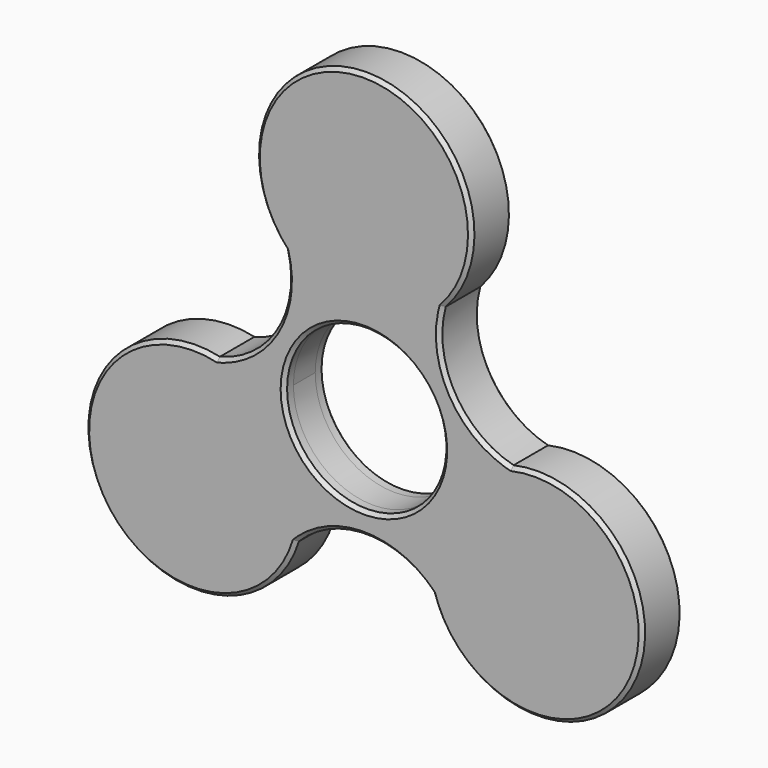
from build123d import *

# Parameters (mm, degrees)
F0_R        = 13.25
F0_R_2      = 11.1
F1_DEPTH    = 3
F2_START    = 1.9
F2_DEPTH    = 1.6
F3_START    = -1.9
F3_DEPTH    = 1.6
F5_D        = 22.2
F6_C1_SIZE  = 0.5
F6_C2_SIZE  = 0.5
F6_C3_SIZE  = 0.4999
F6_C4_SIZE  = 0.4999
F6_C5_SIZE  = 0.4999
F6_C6_SIZE  = 0.4999
F6_C7_SIZE  = 0.4996
F6_C8_SIZE  = 0.5
F6_C9_SIZE  = 0.4999
F6_C10_SIZE = 0.5
F6_C11_SIZE = 0.5
F6_C12_SIZE = 0.4999
F6_C13_SIZE = 0.4996
F6_C14_SIZE = 0.5


# Not quite as in the source:
# - a fillet or chamfer is up to 0.001 mm smaller than in the source, because OpenCascade refuses the exact size


with BuildPart() as f1:
    # F0 (on Front) → F1 (new body, symmetric)
    with BuildSketch(Plane.XZ):
        with BuildLine():
            ThreePointArc((20.4544666255, 0.9003555386), (12.301399045, 7.10221605), (11.0069640816, 17.2639099492))
            ThreePointArc((11.0069640816, 17.2639099492), (0, 42.4544321001), (-11.0069640816, 17.2639099492))
            ThreePointArc((-11.0069640816, 17.2639099492), (-12.301399045, 7.10221605), (-20.4544666255, 0.9003555386))
            ThreePointArc((-20.4544666255, 0.9003555386), (-36.7666167019, -21.22721605), (-9.4475025439, -18.1642654878))
            ThreePointArc((-9.4475025439, -18.1642654878), (0, -14.2044321001), (9.4475025439, -18.1642654878))
            ThreePointArc((9.4475025439, -18.1642654878), (36.7666167019, -21.22721605), (20.4544666255, 0.9003555386))
        make_face()
        with Locations((-23.7762356451, -13.72721605)):
            Circle(F0_R, mode=Mode.SUBTRACT)
        with Locations((23.7762356451, -13.72721605)):
            Circle(F0_R, mode=Mode.SUBTRACT)
        Circle(F0_R_2, mode=Mode.SUBTRACT)
        with Locations((0, 27.4544321001)):
            Circle(F0_R, mode=Mode.SUBTRACT)
    extrude(amount=F1_DEPTH, both=True)

    # F0 (on Front) → F2 (join)
    with BuildSketch(Plane.XZ.offset(F2_START)):
        with BuildLine():
            ThreePointArc((20.4544666255, 0.9003555386), (12.301399045, 7.10221605), (11.0069640816, 17.2639099492))
            ThreePointArc((11.0069640816, 17.2639099492), (0, 42.4544321001), (-11.0069640816, 17.2639099492))
            ThreePointArc((-11.0069640816, 17.2639099492), (-12.301399045, 7.10221605), (-20.4544666255, 0.9003555386))
            ThreePointArc((-20.4544666255, 0.9003555386), (-36.7666167019, -21.22721605), (-9.4475025439, -18.1642654878))
            ThreePointArc((-9.4475025439, -18.1642654878), (0, -14.2044321001), (9.4475025439, -18.1642654878))
            ThreePointArc((9.4475025439, -18.1642654878), (36.7666167019, -21.22721605), (20.4544666255, 0.9003555386))
        make_face()
        with Locations((-23.7762356451, -13.72721605)):
            Circle(F0_R, mode=Mode.SUBTRACT)
        with Locations((23.7762356451, -13.72721605)):
            Circle(F0_R, mode=Mode.SUBTRACT)
        Circle(F0_R_2, mode=Mode.SUBTRACT)
        with Locations((0, 27.4544321001)):
            Circle(F0_R, mode=Mode.SUBTRACT)
        with Locations((-23.7762356451, -13.72721605)):
            Circle(F0_R)
        with Locations((0, 27.4544321001)):
            Circle(F0_R)
        with Locations((23.7762356451, -13.72721605)):
            Circle(F0_R)
        Circle(F0_R_2)
    extrude(amount=F2_DEPTH)

    # F0 (on Front) → F3 (join)
    with BuildSketch(Plane.XZ.offset(F3_START)):
        with BuildLine():
            ThreePointArc((20.4544666255, 0.9003555386), (12.301399045, 7.10221605), (11.0069640816, 17.2639099492))
            ThreePointArc((11.0069640816, 17.2639099492), (0, 42.4544321001), (-11.0069640816, 17.2639099492))
            ThreePointArc((-11.0069640816, 17.2639099492), (-12.301399045, 7.10221605), (-20.4544666255, 0.9003555386))
            ThreePointArc((-20.4544666255, 0.9003555386), (-36.7666167019, -21.22721605), (-9.4475025439, -18.1642654878))
            ThreePointArc((-9.4475025439, -18.1642654878), (0, -14.2044321001), (9.4475025439, -18.1642654878))
            ThreePointArc((9.4475025439, -18.1642654878), (36.7666167019, -21.22721605), (20.4544666255, 0.9003555386))
        make_face()
        with Locations((-23.7762356451, -13.72721605)):
            Circle(F0_R, mode=Mode.SUBTRACT)
        with Locations((23.7762356451, -13.72721605)):
            Circle(F0_R, mode=Mode.SUBTRACT)
        Circle(F0_R_2, mode=Mode.SUBTRACT)
        with Locations((0, 27.4544321001)):
            Circle(F0_R, mode=Mode.SUBTRACT)
        with Locations((0, 27.4544321001)):
            Circle(F0_R)
        with Locations((-23.7762356451, -13.72721605)):
            Circle(F0_R)
        with Locations((23.7762356451, -13.72721605)):
            Circle(F0_R)
        Circle(F0_R_2)
    extrude(amount=-F3_DEPTH)

    # F5 (through all)
    with Locations(Plane.XZ.offset(3.5)):
        with Locations((0, 0)):
            Hole(F5_D / 2)

    # F6: chamfer of 0.5 on 14 edges, made by hand

    # F6_c1
    f6_c1_edges = [f1.edges().sort_by_distance(p)[0] for p in [
        (12.301399045, 3.5, 7.10221605),
    ]]
    chamfer(f6_c1_edges, length=F6_C1_SIZE)

    # F6_c2
    f6_c2_edges = [f1.edges().sort_by_distance(p)[0] for p in [
        (12.301399045, -3.5, 7.10221605),
    ]]
    chamfer(f6_c2_edges, length=F6_C2_SIZE)

    # F6_c3 (size 0.5 in the source; OpenCascade refuses exactly that, so slightly less here)
    f6_c3_edges = [f1.edges().sort_by_distance(p)[0] for p in [
        (36.7666167019, 3.5, -21.22721605),
    ]]
    chamfer(f6_c3_edges, length=F6_C3_SIZE)

    # F6_c4 (size 0.5 in the source; OpenCascade refuses exactly that, so slightly less here)
    f6_c4_edges = [f1.edges().sort_by_distance(p)[0] for p in [
        (0, 3.5, 42.4544321001),
    ]]
    chamfer(f6_c4_edges, length=F6_C4_SIZE)

    # F6_c5 (size 0.5 in the source; OpenCascade refuses exactly that, so slightly less here)
    f6_c5_edges = [f1.edges().sort_by_distance(p)[0] for p in [
        (0, 3.5, -14.2044321001),
    ]]
    chamfer(f6_c5_edges, length=F6_C5_SIZE)

    # F6_c6 (size 0.5 in the source; OpenCascade refuses exactly that, so slightly less here)
    f6_c6_edges = [f1.edges().sort_by_distance(p)[0] for p in [
        (-12.301399045, 3.5, 7.10221605),
    ]]
    chamfer(f6_c6_edges, length=F6_C6_SIZE)

    # F6_c7 (size 0.5 in the source; OpenCascade refuses exactly that, so slightly less here)
    f6_c7_edges = [f1.edges().sort_by_distance(p)[0] for p in [
        (-36.7666167019, 3.5, -21.22721605),
    ]]
    chamfer(f6_c7_edges, length=F6_C7_SIZE)

    # F6_c8
    f6_c8_edges = [f1.edges().sort_by_distance(p)[0] for p in [
        (-11.1, 3.5, 0),
    ]]
    chamfer(f6_c8_edges, length=F6_C8_SIZE)

    # F6_c9 (size 0.5 in the source; OpenCascade refuses exactly that, so slightly less here)
    f6_c9_edges = [f1.edges().sort_by_distance(p)[0] for p in [
        (0, -3.5, 42.4544321001),
    ]]
    chamfer(f6_c9_edges, length=F6_C9_SIZE)

    # F6_c10
    f6_c10_edges = [f1.edges().sort_by_distance(p)[0] for p in [
        (36.7666167019, -3.5, -21.22721605),
    ]]
    chamfer(f6_c10_edges, length=F6_C10_SIZE)

    # F6_c11
    f6_c11_edges = [f1.edges().sort_by_distance(p)[0] for p in [
        (0, -3.5, -14.2044321001),
    ]]
    chamfer(f6_c11_edges, length=F6_C11_SIZE)

    # F6_c12 (size 0.5 in the source; OpenCascade refuses exactly that, so slightly less here)
    f6_c12_edges = [f1.edges().sort_by_distance(p)[0] for p in [
        (-12.301399045, -3.5, 7.10221605),
    ]]
    chamfer(f6_c12_edges, length=F6_C12_SIZE)

    # F6_c13 (size 0.5 in the source; OpenCascade refuses exactly that, so slightly less here)
    f6_c13_edges = [f1.edges().sort_by_distance(p)[0] for p in [
        (-36.7666167019, -3.5, -21.22721605),
    ]]
    chamfer(f6_c13_edges, length=F6_C13_SIZE)

    # F6_c14
    f6_c14_edges = [f1.edges().sort_by_distance(p)[0] for p in [
        (-11.1, -3.5, 0),
    ]]
    chamfer(f6_c14_edges, length=F6_C14_SIZE)


solid = f1.part
